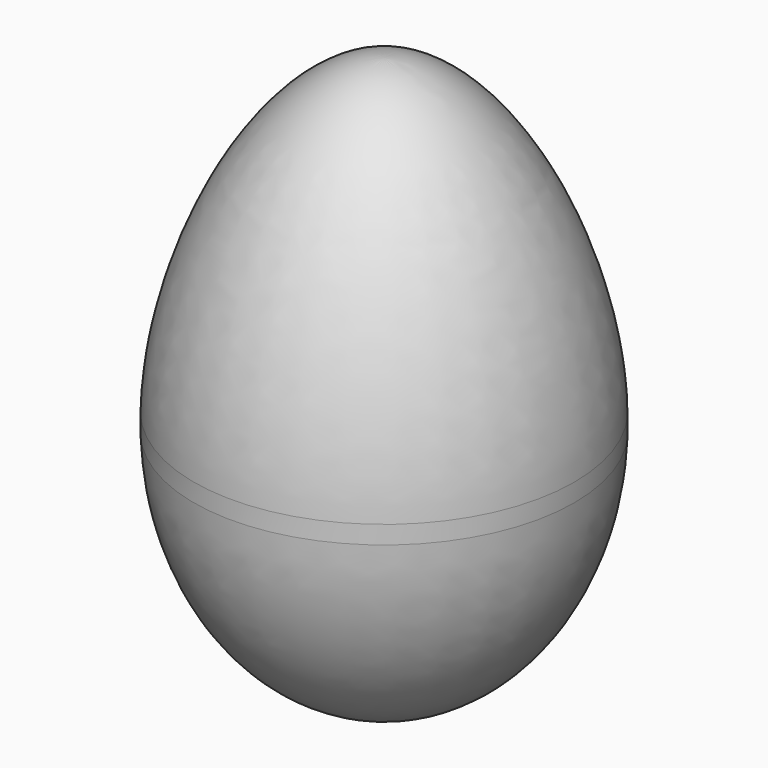
from build123d import *

# Parameters (mm, degrees)
F2_T          = -3
F5_T          = -3
F4_R          = 22.2704803826
F4_R_2        = 19.2704803826
F6_DEPTH      = 5
F7_DEPTH      = 4
F7_DEPTH_BACK = 16.0339293929
F8_R          = 19.2704803826
F14_DEPTH     = 15.001


with BuildPart() as f1:
    # F0 (on Front) → F1 (revolve)
    with BuildSketch(Plane.XZ):
        with BuildLine():
            Line((25.2704803826, -2.4096544784), (25.2704803826, 0))
            Line((25.2704803826, 0), (0, 0))
            Line((0, 0), (0, -33.6620144546))
            add(Edge.make_bspline(
                [(25.2704803826, -2.4096544784), (24.7897152524, -19.8217053945), (13.7113224277, -33.6620144546), (0, -33.6620144546)],
                knots=[0.5294301915, 0.5294301915, 0.5294301915, 0.5294301915, 1, 1, 1, 1], degree=3))
        make_face()
    revolve(axis=Axis((0, 0, 3.8379855454), (0, 0, 1)))

    # F2
    f2_openings = [f1.faces().sort_by_distance(p)[0] for p in [
        (0, 0, 0),
    ]]
    offset(amount=F2_T, openings=f2_openings)

    # F4 (on face) → F7 (join, two sides)
    with BuildSketch(Plane(origin=(0, 0, 0), x_dir=(1, 0, 0), z_dir=(0, 0, -1))) as f7_sk:
        Circle(F4_R)
        Circle(F4_R_2, mode=Mode.SUBTRACT)
    extrude(amount=-F7_DEPTH)
    extrude(f7_sk.sketch, amount=F7_DEPTH_BACK)


with BuildPart() as f3:
    # F0 (on Front) → F3 (revolve)
    with BuildSketch(Plane.XZ):
        with BuildLine():
            add(Edge.make_bspline(
                [(0, 41.3379855454), (12.3329152107, 41.3379855454), (24.7585030056, 19.104272726), (25.2704803826, 0)],
                knots=[0, 0, 0, 0, 0.507909238, 0.507909238, 0.507909238, 0.507909238], degree=3))
            Line((0, 41.3379855454), (0, 0))
            Line((0, 0), (25.2704803826, 0))
        make_face()
    revolve(axis=Axis((0, 0, 3.8379855454), (0, 0, 1)))

    # F5
    f5_openings = [f3.faces().sort_by_distance(p)[0] for p in [
        (0, 0, 0),
    ]]
    offset(amount=F5_T, openings=f5_openings)

    # F4 (on face) → F6 (cut)
    with BuildSketch(Plane(origin=(0, 0, 0), x_dir=(1, 0, 0), z_dir=(0, 0, -1))):
        Circle(F4_R)
        Circle(F4_R_2, mode=Mode.SUBTRACT)
        Circle(F4_R_2)
    extrude(amount=-F6_DEPTH, mode=Mode.SUBTRACT)

    # F8 (on face) → F9 (join, up to the next surface of F3)
    with BuildSketch(Plane(origin=(0, 0, 5), x_dir=(1, 0, 0), z_dir=(0, 0, -1))):
        with BuildLine():
            add(Edge.make_bspline(
                [(21.8537308611, 0), (21.8537309387, 2.1449379384), (21.6131301275, 4.2913342313), (21.1313607898, 6.4054317488), (20.4142007343, 8.4558388096), (19.4714527317, 10.4128042822), (18.3172224176, 12.2483593456), (16.9696215019, 13.9362211797), (13.9240999767, 16.9817427136), (12.2213448637, 18.3387765002), (10.3687100045, 19.4991267243), (8.393153203, 20.4442919919), (6.3233537078, 21.1598981104), (4.1898178598, 21.6360213556), (2.0247270979, 21.8668842305), (-2.2650634285, 21.8399303148), (-4.3927300328, 21.589786643), (-6.4873906464, 21.1025341797), (-8.5184305526, 20.3839469868), (-10.4568411063, 19.4437049015), (-12.2753518345, 18.2956470716), (-13.9483428566, 16.9574998167), (-16.9696215019, 13.9362211797), (-18.3172224176, 12.2483593456), (-19.4714527316, 10.4128042821), (-20.4142007344, 8.4558388097), (-21.1313607897, 6.4054317487), (-21.6131301275, 4.2913342314), (-21.8537309387, 2.1449379384), (-21.8537309387, -2.1449379384), (-21.6131301275, -4.2913342313), (-21.1313607896, -6.4054317489), (-20.4142007345, -8.4558388095), (-19.4714527315, -10.4128042823), (-18.3172224177, -12.2483593456), (-16.9696215019, -13.9362211797), (-13.9362211789, -16.9696215026), (-12.2483593451, -18.3172224185), (-10.4128042814, -19.4714527301), (-8.4558388093, -20.4142007352), (-6.4054317459, -21.1313607834), (-4.2913342328, -21.6131301361), (-2.1449379385, -21.8537309388), (2.1449379385, -21.8537309388), (4.2913342327, -21.6131301361), (6.4054317461, -21.1313607834), (8.455838809, -20.4142007353), (10.4128042816, -19.47145273), (12.248359345, -18.3172224186), (13.936221179, -16.9696215026), (16.9696215019, -13.9362211797), (18.3172224176, -12.2483593456), (19.4714527317, -10.4128042822), (20.4142007342, -8.4558388096), (21.1313607899, -6.4054317488), (21.6131301274, -4.2913342314), (21.8537309387, -2.1449379384), (21.8537308611, 0)],
                knots=[0, 0, 0, 0, 0, 0, 0, 0, 0, 0.1250000049, 0.1250000049, 0.1250000049, 0.1250000049, 0.1250000049, 0.1250000049, 0.1250000049, 0.25099899, 0.25099899, 0.25099899, 0.25099899, 0.25099899, 0.25099899, 0.25099899, 0.3749999756, 0.3749999756, 0.3749999756, 0.3749999756, 0.3749999756, 0.3749999756, 0.3749999756, 0.4999999805, 0.4999999805, 0.4999999805, 0.4999999805, 0.4999999805, 0.4999999805, 0.4999999805, 0.6249999853, 0.6249999853, 0.6249999853, 0.6249999853, 0.6249999853, 0.6249999853, 0.6249999853, 0.7499999902, 0.7499999902, 0.7499999902, 0.7499999902, 0.7499999902, 0.7499999902, 0.7499999902, 0.8749999951, 0.8749999951, 0.8749999951, 0.8749999951, 0.8749999951, 0.8749999951, 0.8749999951, 1, 1, 1, 1, 1, 1, 1, 1, 1], degree=8))
        make_face()
        Circle(F8_R, mode=Mode.SUBTRACT)
    extrude(until=Until.NEXT, dir=(0, 0, 1))


with BuildPart() as f11:
    # F10 (on Front) → F11 (revolve)
    with BuildSketch(Plane.XZ):
        Polygon((11.6602540378, -15), (4.443375673, -2.5), (2.5, -2.5), (2.5, -15), align=None)
    revolve(axis=Axis((0, 0, -5.9531112202), (0, 0, 1)))


with BuildPart() as f12:
    # F10 (on Front) → F12 (revolve)
    with BuildSketch(Plane.XZ):
        Polygon((19.2704803826, 0), (3, 0), (4.443375673, -2.5), (11.6602540378, -15), (19.2704803826, -15), align=None)
    revolve(axis=Axis((0, 0, -5.9531112202), (0, 0, 1)))

    # F13 (on face) → F14 (cut, through all)
    with BuildSketch(Plane.XY):
        with BuildLine():
            ThreePointArc((-1.5, 2.5980762114), (0, 3), (1.5, 2.5980762114))
            Line((1.5, 2.5980762114), (1.5, 19.2120122365))
            ThreePointArc((1.5, 19.2120122365), (0, 19.2704803826), (-1.5, 19.2120122365))
            Line((-1.5, 19.2120122365), (-1.5, 2.5980762114))
        make_face()
        with BuildLine():
            Line((-15.8880906547, -10.9050442239), (-1.5, -2.5980762114))
            ThreePointArc((-1.5, -2.5980762114), (-2.5980762114, -1.5), (-3, 0))
            Line((-3, 0), (-17.3880906547, -8.3069680126))
            ThreePointArc((-17.3880906547, -8.3069680126), (-16.6887255545, -9.6352401913), (-15.8880906547, -10.9050442239))
        make_face()
        with BuildLine():
            Line((17.3880906547, -8.3069680126), (3, 0))
            ThreePointArc((3, 0), (2.5980762114, -1.5), (1.5, -2.5980762114))
            Line((1.5, -2.5980762114), (15.8880906547, -10.9050442239))
            ThreePointArc((15.8880906547, -10.9050442239), (16.6887255545, -9.6352401913), (17.3880906547, -8.3069680126))
        make_face()
    extrude(amount=-F14_DEPTH, mode=Mode.SUBTRACT)


solid = Compound([f1.part, f3.part, f11.part, f12.part])
